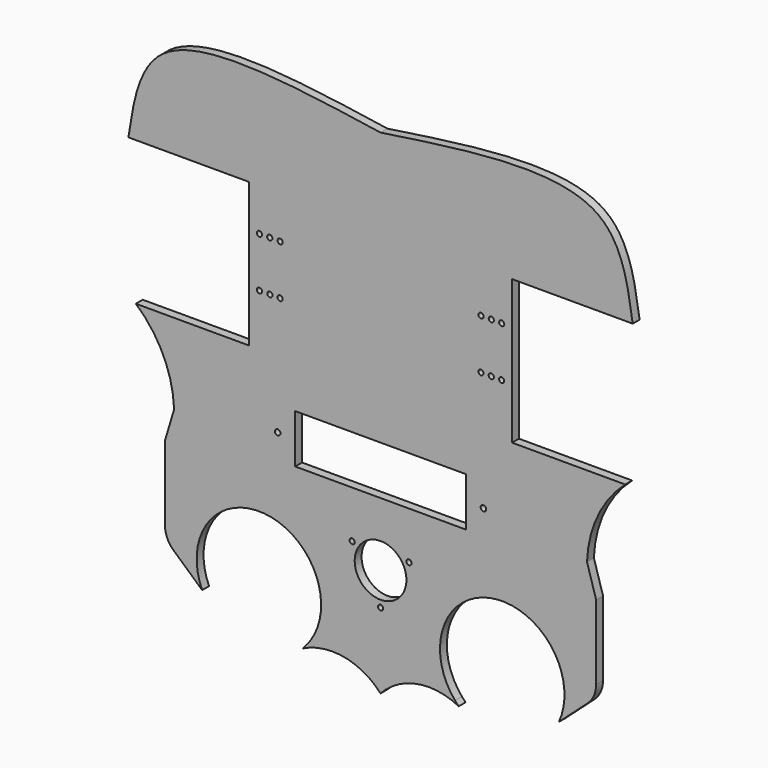
from build123d import *

# Parameters (mm, degrees)
F0_R     = 1.6
F0_R_2   = 1.5
F1_DEPTH = 5


with BuildPart() as f1:
    # F0 (on Front) → F1 (new body)
    with BuildSketch(Plane.XZ):
        with BuildLine():
            Line((0, -105.5724638663), (0, -98.9320270717))
            Line((0, -98.9320270717), (0, -87.6365141757))
            Line((0, -87.6365141757), (-49.5, -87.6365141757))
            Line((-49.5, -87.6365141757), (-49.5, -59.3522429283))
            Line((-49.5, -59.3522429283), (0, -59.3522429283))
            Line((0, -59.3522429283), (0, 98.9320270717))
            add(Edge.make_bspline(
                [(-146.2381845713, 48.9320270717), (-143.2091262015, 68.9096288331), (-135.5852518703, 119.1915008468), (-50.9865840375, 106.55056484), (0, 98.9320270717)],
                knots=[0, 0, 0, 0, 0.3973122114, 1, 1, 1, 1], degree=3))
            Line((-146.2381845713, 48.9320270717), (-125, 48.9320270717))
            Line((-125, 48.9320270717), (-76.2381845713, 48.9320270717))
            Line((-76.2381845713, 48.9320270717), (-76.2381845713, -34.5724638663))
            Line((-76.2381845713, -34.5724638663), (-141.8916900928, -34.5724638663))
            ThreePointArc((-141.8916900928, -34.5724638663), (-125.9898971587, -55.6502114599), (-119.7161859861, -81.2974142364))
            Line((-119.7161859861, -81.2974142364), (-125, -98.9320270717))
            Line((-125, -98.9320270717), (-125, -142.2410042337))
            ThreePointArc((-125, -142.2410042337), (-123.6989053151, -148.3516501216), (-120.0213342443, -153.4022254914))
            Line((-120.0213342443, -153.4022254914), (-103.4289673704, -168.3000265931))
            ThreePointArc((-103.4289673704, -168.3000265931), (-65.4068612322, -117.6788317827), (-43.2242829938, -176.9757047349))
            ThreePointArc((-43.2242829938, -176.9757047349), (-44.2540337338, -178.1193368484), (-45.3315999714, -179.2180324392))
            ThreePointArc((-45.3315999714, -179.2180324392), (-21.2811980726, -175.6350274134), (0, -187.3981207609))
            Line((0, -187.3981207609), (0, -179.2180324392))
            Line((0, -179.2180324392), (0, -145.0724638663))
            ThreePointArc((0, -145.0724638663), (-1.0813916472, -144.6119791886), (-1.4988309156, -143.51325334))
            ThreePointArc((-1.4988309156, -143.51325334), (-16.4544826719, -134.0724638663), (-17.1526203097, -116.4000947784))
            ThreePointArc((-17.1526203097, -116.4000947784), (-17.7535207776, -114.3224638663), (-15.6537893941, -113.8040434806))
            ThreePointArc((-15.6537893941, -113.8040434806), (-8.843076746, -107.755805647), (0, -105.5724638663))
        make_face()
        with Locations((-59.6421356237, -73.494378552)):
            Circle(F0_R, mode=Mode.SUBTRACT)
        with BuildLine():
            ThreePointArc((-70.2381845713, -6.0724638663), (-71.298844743, -3.5118036945), (-68.7381845713, -4.5724638663))
            ThreePointArc((-68.7381845713, -4.5724638663), (-69.1775243995, -5.6331240381), (-70.2381845713, -6.0724638663))
        make_face(mode=Mode.SUBTRACT)
        with Locations((-64.1868777356, -4.5724638663)):
            Circle(F0_R_2, mode=Mode.SUBTRACT)
        with Locations((-58.2381845713, -4.5724638663)):
            Circle(F0_R_2, mode=Mode.SUBTRACT)
        with Locations((-70.2381845713, 24.4275361337)):
            Circle(F0_R_2, mode=Mode.SUBTRACT)
        with Locations((-64.2381845713, 24.4275361337)):
            Circle(F0_R_2, mode=Mode.SUBTRACT)
        with Locations((-58.2381845713, 24.4275361337)):
            Circle(F0_R_2, mode=Mode.SUBTRACT)
        with BuildLine():
            Line((0, -87.6365141757), (0, -98.9320270717))
            Line((0, -98.9320270717), (0, -105.5724638663))
            ThreePointArc((0, -105.5724638663), (8.843076746, -107.755805647), (15.6537893941, -113.8040434806))
            ThreePointArc((15.6537893941, -113.8040434806), (17.178692615, -113.7588733828), (17.9544826719, -115.0724638663))
            ThreePointArc((17.9544826719, -115.0724638663), (17.738462122, -115.8479616237), (17.1526203097, -116.4000947784))
            ThreePointArc((17.1526203097, -116.4000947784), (18.5324011651, -120.3831790756), (19, -124.5724638663))
            ThreePointArc((19, -124.5724638663), (13.9548878067, -137.4666915013), (1.4988309156, -143.51325334))
            ThreePointArc((1.4988309156, -143.51325334), (1.4997077004, -143.542852833), (1.5, -143.5724638663))
            ThreePointArc((1.5, -143.5724638663), (1.0606601718, -144.6331240381), (0, -145.0724638663))
            Line((0, -145.0724638663), (0, -179.2180324392))
            Line((0, -179.2180324392), (0, -187.3981207609))
            ThreePointArc((0, -187.3981207609), (21.2811980726, -175.6350274134), (45.3315999714, -179.2180324392))
            ThreePointArc((45.3315999714, -179.2180324392), (44.2540337338, -178.1193368484), (43.2242829938, -176.9757047349))
            ThreePointArc((43.2242829938, -176.9757047349), (65.4068612322, -117.6788317827), (103.4289673704, -168.3000265931))
            Line((103.4289673704, -168.3000265931), (120.0213342443, -153.4022254914))
            ThreePointArc((120.0213342443, -153.4022254914), (123.6989053151, -148.3516501216), (125, -142.2410042337))
            Line((125, -142.2410042337), (125, -98.9320270717))
            Line((125, -98.9320270717), (119.7161859861, -81.2974142364))
            ThreePointArc((119.7161859861, -81.2974142364), (125.9898971587, -55.6502114599), (141.8916900928, -34.5724638663))
            Line((141.8916900928, -34.5724638663), (76.2381845713, -34.5724638663))
            Line((76.2381845713, -34.5724638663), (76.2381845713, 48.9320270717))
            Line((76.2381845713, 48.9320270717), (125, 48.9320270717))
            Line((125, 48.9320270717), (146.2381845713, 48.9320270717))
            add(Edge.make_bspline(
                [(146.2381845713, 48.9320270717), (143.2091262015, 68.9096288331), (135.5852518703, 119.1915008468), (50.9865840375, 106.55056484), (0, 98.9320270717)],
                knots=[0, 0, 0, 0, 0.3973122114, 1, 1, 1, 1], degree=3))
            Line((0, 98.9320270717), (0, -59.3522429283))
            Line((0, -59.3522429283), (49.5, -59.3522429283))
            Line((49.5, -59.3522429283), (49.5, -87.6365141757))
            Line((49.5, -87.6365141757), (0, -87.6365141757))
        make_face()
        with Locations((59.6421356237, -73.494378552)):
            Circle(F0_R, mode=Mode.SUBTRACT)
        with Locations((58.2381845713, -4.5724638663)):
            Circle(F0_R_2, mode=Mode.SUBTRACT)
        with Locations((64.1868777356, -4.5724638663)):
            Circle(F0_R_2, mode=Mode.SUBTRACT)
        with Locations((70.2381845713, -4.5724638663)):
            Circle(F0_R_2, mode=Mode.SUBTRACT)
        with Locations((58.2381845713, 24.4275361337)):
            Circle(F0_R_2, mode=Mode.SUBTRACT)
        with Locations((64.2381845713, 24.4275361337)):
            Circle(F0_R_2, mode=Mode.SUBTRACT)
        with Locations((70.2381845713, 24.4275361337)):
            Circle(F0_R_2, mode=Mode.SUBTRACT)
        with BuildLine():
            ThreePointArc((15.6537893941, -113.8040434806), (8.843076746, -107.755805647), (0, -105.5724638663))
            Line((0, -105.5724638663), (0, -109.5724638663))
            ThreePointArc((0, -109.5724638663), (10.6066017178, -113.9658621485), (15, -124.5724638663))
            ThreePointArc((15, -124.5724638663), (10.6066017178, -135.1790655841), (0, -139.5724638663))
            Line((0, -139.5724638663), (0, -142.0724638663))
            ThreePointArc((0, -142.0724638663), (1.0395153223, -142.4910722191), (1.4988309156, -143.51325334))
            ThreePointArc((1.4988309156, -143.51325334), (13.9548878067, -137.4666915013), (19, -124.5724638663))
            ThreePointArc((19, -124.5724638663), (18.5324011651, -120.3831790756), (17.1526203097, -116.4000947784))
            ThreePointArc((17.1526203097, -116.4000947784), (15.1554445662, -115.8224638663), (15.6537893941, -113.8040434806))
        make_face()
        with BuildLine():
            Line((0, -109.5724638663), (0, -105.5724638663))
            ThreePointArc((0, -105.5724638663), (-8.843076746, -107.755805647), (-15.6537893941, -113.8040434806))
            ThreePointArc((-15.6537893941, -113.8040434806), (-15.1408921884, -114.3482539232), (-14.9544826719, -115.0724638663))
            ThreePointArc((-14.9544826719, -115.0724638663), (-15.6789849146, -116.3564433165), (-17.1526203097, -116.4000947784))
            ThreePointArc((-17.1526203097, -116.4000947784), (-16.4544826719, -134.0724638663), (-1.4988309156, -143.51325334))
            ThreePointArc((-1.4988309156, -143.51325334), (-1.0395153223, -142.4910722191), (0, -142.0724638663))
            Line((0, -142.0724638663), (0, -139.5724638663))
            ThreePointArc((0, -139.5724638663), (-15, -124.5724638663), (0, -109.5724638663))
        make_face()
    extrude(amount=F1_DEPTH)


solid = f1.part
